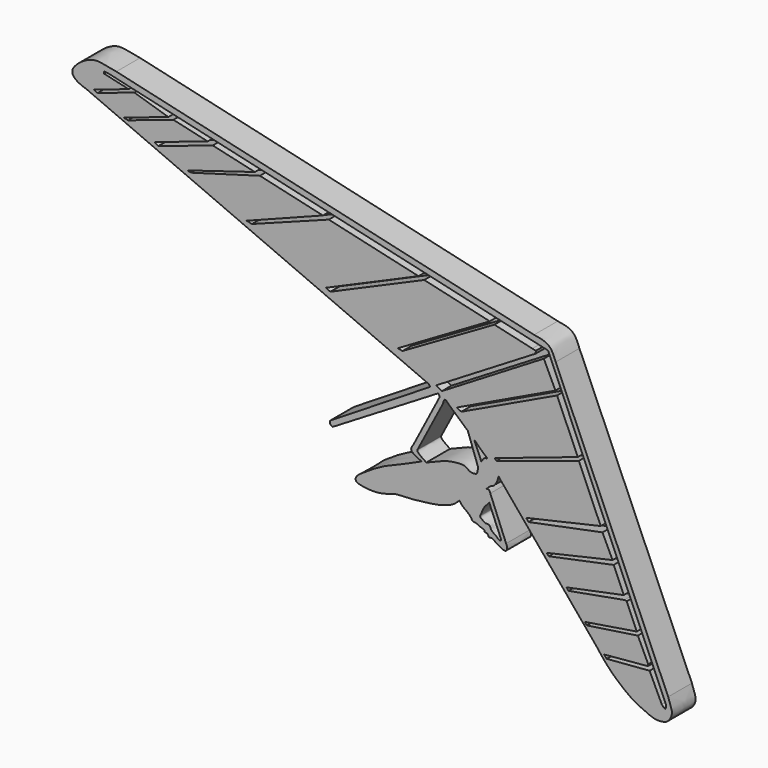
from build123d import *

# Parameters (mm, degrees)
F1_DEPTH = 3
F2_DEPTH = 5


with BuildPart() as f1:
    # F0 (on Front) → F1 (new body)
    with BuildSketch(Plane.XZ):
        with BuildLine():
            add(Edge.make_bspline(
                [(-3.958843658, -0.272790711), (-4.2719665821, 0.0142837838), (-4.643623801, 0.3451680177), (-5.0374746802, 0.6923990015)],
                knots=[0.7600893092, 0.7600893092, 0.7600893092, 0.7600893092, 0.7909645416, 0.7909645416, 0.7909645416, 0.7909645416], degree=3))
            Line((-5.0374746802, 0.6923990015), (-3.2803696069, -4.2355656273))
            add(Edge.make_bspline(
                [(-3.2803696069, -4.2355656273), (-3.1553498333, -3.8691138278), (-2.9633792204, -3.454910973), (-2.7671998453, -3.1178165413)],
                knots=[0.4986063056, 0.4986063056, 0.4986063056, 0.4986063056, 0.5447587412, 0.5447587412, 0.5447587412, 0.5447587412], degree=3))
            Line((-2.7671998453, -3.1178165413), (-3.958843658, -0.272790711))
        make_face()
    extrude(amount=F1_DEPTH)



with BuildPart() as f1b:
    # F0 (on Front) → F1, piece 2 (new body)
    with BuildSketch(Plane.XZ):
        Polygon((7.5457381318, 17.2318940768), (-65.6217709184, 34.0295992792), (-66.3976059657, 34.1109745204), (-66.3976059657, 33.7685608692), (-63.0448907614, 32.9988487065), (-62.215026468, 32.8109674156), (-68.1188135161, 30.8244369209), (-67.4496538422, 30.5345711273), (-61.2546354532, 32.6190963387), (-55.5289892554, 30.8500090748), (-63.0566432516, 28.3170731652), (-62.3126912516, 28.1462775956), (-54.6743792028, 30.7164481809), (-48.8941353204, 29.3894270209), (-57.8368790448, 26.3803359121), (-57.2307138925, 25.9741354846), (-48.0405491438, 29.066479835), (-40.9353561699, 27.43527852), (-52.3144661485, 23.9721520054), (-51.701374352, 23.8313991576), (-40.0919642747, 27.1510338508), (-29.472887516, 24.7131194919), (-42.3169331915, 19.753197379), (-41.4403453469, 19.5519514382), (-28.4778410115, 24.4221122192), (-13.3526945596, 20.9497000169), (-28.9905350655, 14.1369793564), (-28.2068449965, 13.8057659517), (-12.3952388368, 20.6941886798), (-1.3400092721, 18.1561429054), (-16.8327485305, 9.1245940536), (-16.0704851151, 8.9495945722), (-0.5562102706, 17.907858254), (5.831264226, 16.4414298492), (6.4167166129, 16.3070224226), (6.3947961883, 15.8712696639), (-10.4206494301, 5.6898728398), (-9.4167995289, 5.1668914956), (-6.9013429763, 6.6899472585), (7.7697090081, 15.5729590722), (9.7222536882, 11.4739608713), (-6.8918203924, 3.5598998321), (-6.1443895223, 3.1705065566), (10.0013106788, 10.8408021783), (13.4894661484, 2.8341303049), (-0.4957623773, -1.8716767838), (-0.2358101605, -2.1840042965), (13.6655064476, 2.3245441099), (17.3558875858, -6.1463142333), (4.8005964737, -9.0149185256), (5.2074594302, -9.5037564234), (17.6518484829, -6.989151013), (19.3531792489, -10.5476134987), (8.2439421993, -13.0858266553), (8.5738468794, -13.4822006867), (19.5388207109, -11.2054196425), (21.2328508375, -15.1317070768), (11.5879603013, -17.1178100351), (11.9304004935, -17.5292452396), (21.3820858062, -15.8089878546), (21.7298547311, -15.8888282094), (23.4441608069, -19.8238266231), (14.6837355114, -21.2355394273), (15.0275071961, -21.6485743941), (23.6202347902, -20.3643494816), (25.3650247929, -24.0533517272), (25.3243371723, -24.3517288537), (17.9191976664, -25.0162927033), (18.3667614934, -25.5181060703), (25.5955885974, -24.934917462), (27.6435296861, -29.2613615812), (28.0233658055, -29.6726883891), (28.2402802137, -29.7224873276), (28.321655455, -29.5868625463), (28.375904995, -29.1121748806), (8.4721240049, 17.0192155669), align=None)
    extrude(amount=F1_DEPTH)


with BuildPart() as f1_1:
    add(f1.part)

    add(f1b.part)  # F2 merges F1b
    # F0 (on Front) → F2 (join)
    with BuildSketch(Plane.XZ):
        with BuildLine():
            add(Edge.make_bspline(
                [(-69.2230314016, 30.4545033723), (-69.9181913826, 30.689063994), (-71.1847424521, 31.1164231839), (-72.3137756024, 32.8148190164), (-68.6665327756, 35.5511735287), (-66.3988625608, 35.128581332), (-64.9777753981, 34.86736873), (-64.2862692475, 34.7402617335)],
                knots=[0, 0, 0, 0, 0.1908374714, 0.347697523, 0.607024674, 0.8087767858, 1, 1, 1, 1], degree=3))
            Line((-69.2230314016, 30.4545033723), (-11.5922411632, 5.4900660326))
            Line((-11.5922411632, 5.4900660326), (-11.3857872784, 5.1581566222))
            Line((-11.3857872784, 5.1581566222), (-28.2431393862, -5.327432882))
            add(Edge.make_bspline(
                [(-27.8076659888, -6.1177369207), (-27.9722888528, -6.0516858021), (-28.3106523524, -5.9159252697), (-28.266044387, -5.5270896206), (-28.2431393862, -5.327432882)],
                knots=[0, 0, 0, 0, 0.4865266622, 1, 1, 1, 1], degree=3))
            Line((-27.8076659888, -6.1177369207), (-10.2219458664, 4.530044831))
            Line((-10.2219458664, 4.530044831), (-10.0369686261, 4.6426397748))
            Line((-10.0369686261, 4.6426397748), (-9.7684441134, 4.2014927603))
            Line((-9.7684441134, 4.2014927603), (-14.1773857176, -4.261362832))
            add(Edge.make_bspline(
                [(-12.7947209403, -6.3626165502), (-13.0334271505, -6.2805139246), (-13.5184917895, -6.1136767049), (-14.220189292, -5.6478018131), (-14.531709537, -5.4241327279), (-14.6556915825, -4.9871926824), (-14.3576112479, -4.5348553382), (-14.1773857176, -4.261362832)],
                knots=[0, 0, 0, 0, 0.2243166321, 0.4558241953, 0.6092440098, 0.7637408531, 1, 1, 1, 1], degree=3))
            add(Edge.make_bspline(
                [(-6.4495992847, -10.100312531), (-6.7441156637, -10.3927897932), (-7.3501218579, -10.9946002362), (-8.7041020642, -11.5541608562), (-10.0684563701, -11.9645084942), (-12.7031852773, -12.3310429211), (-15.730053764, -12.6261937319), (-17.2652343001, -12.5335072447), (-19.3279665226, -13.3871483962), (-21.2038717611, -13.4796836708), (-22.611676204, -13.359816129), (-24.0173983346, -13.0521736195), (-23.9696116255, -12.1275719541), (-22.621292381, -11.1758610844), (-21.1033539259, -10.2092903874), (-18.9497480388, -8.9271541368), (-15.0096411192, -7.423031309), (-13.4627235854, -6.6824293681), (-12.7947209403, -6.3626165502)],
                knots=[0, 0, 0, 0, 0.0512015152, 0.1053538533, 0.1595452957, 0.2346660875, 0.3143966362, 0.3709639138, 0.4378890012, 0.5004742743, 0.5561906401, 0.6069183652, 0.6431262878, 0.7002532752, 0.7618580709, 0.8346312867, 0.9285891229, 1, 1, 1, 1], degree=3))
            add(Edge.make_bspline(
                [(1.4102349523, -13.9269949868), (1.4749419549, -14.0812995688), (1.5951120677, -14.367865137), (1.6227209485, -14.8859002425), (1.1354026117, -15.1691694816), (0.4498641561, -14.7477156812), (-0.6640591092, -14.1716147874), (-0.964249599, -13.8580024095), (-1.4951999347, -14.0043591013), (-1.5685727115, -13.7207736017), (-1.8192065789, -13.3827013104), (-2.2717811663, -13.4351631175), (-2.2071364287, -13.010901004), (-2.8066379941, -13.0058014509), (-3.38081436, -12.5444686941), (-4.3147683124, -12.4988410556), (-4.4675737318, -11.9207481219), (-5.4031459263, -11.1189747582), (-5.9573777545, -10.8137728678), (-6.2798680182, -10.3410311014), (-6.4495992847, -10.100312531)],
                knots=[0, 0, 0, 0, 0.0514729921, 0.1014592787, 0.149221469, 0.2145230836, 0.2975211894, 0.3450601704, 0.3934120742, 0.4289236754, 0.47548306, 0.5189702295, 0.5567780208, 0.6075660577, 0.6723047127, 0.7388670026, 0.792399205, 0.8726835822, 0.9325882721, 1, 1, 1, 1], degree=3))
            Line((1.4102349523, -13.9269949868), (-1.2545015197, -7.343289908))
            add(Edge.make_bspline(
                [(0.4007980169, -4.7088088468), (0.310436534, -4.5520931225), (0.1140061778, -4.2114200332), (0.023724046, -5.001467346), (-0.2868815855, -5.5909447621), (-0.7107437927, -6.1131980187), (-1.2324368171, -6.2077198768), (-1.69872509, -6.6995691869), (-1.9511121659, -6.9357491466), (-1.4844889637, -6.73770814), (-1.3402720814, -7.1174467598), (-1.2545015197, -7.343289908)],
                knots=[0, 0, 0, 0, 0.0984772063, 0.2140725462, 0.3524954365, 0.4780678856, 0.5924230264, 0.7267704517, 0.7940044635, 0.8774876243, 1, 1, 1, 1], degree=3))
            Line((0.4007980169, -4.7088088468), (16.64548181, -24.2264792323))
            add(Edge.make_bspline(
                [(28.7290737033, -27.7940165251), (28.9117644633, -28.3099578967), (29.2391090465, -29.2344196111), (29.4945885215, -30.1956884574), (28.7931095169, -31.4654049104), (28.0013465038, -31.7902524263), (26.5785107763, -31.9730053275), (24.6056557437, -31.0893777432), (22.4111262769, -30.1005694812), (18.7903829231, -27.053984243), (17.329002501, -25.1275269155), (16.64548181, -24.2264792323)],
                knots=[0, 0, 0, 0, 0.0993022054, 0.1779293, 0.2692963707, 0.341902863, 0.4346793497, 0.5499136078, 0.6756716751, 0.8483043037, 1, 1, 1, 1], degree=3))
            Line((28.7290737033, -27.7940165251), (9.7696268931, 15.7252792269))
            add(Edge.make_bspline(
                [(6.1201294884, 18.5764487833), (6.794057073, 18.470796703), (8.0256136154, 18.2777247564), (9.1324021938, 17.3905574188), (9.5470495227, 16.3069472653), (9.7696268931, 15.7252792269)],
                knots=[0, 0, 0, 0, 0.3589004256, 0.6558659674, 1, 1, 1, 1], degree=3))
            Line((6.1201294884, 18.5764487833), (-64.2862692475, 34.7402617335))
        make_face()
        with BuildLine():
            add(Edge.make_bspline(
                [(0.4983769031, -13.4383020923), (0.5218137706, -13.5645244168), (0.5644444565, -13.7941175684), (0.2328431432, -13.8910706937), (-0.1654042371, -13.3790911879), (-0.7574425902, -13.0664055933), (-1.2446881019, -12.6109943897), (-1.3271120749, -11.9540819736), (-2.10476145, -12.1123359576), (-2.3607071265, -11.8356934552), (-3.1441042369, -11.4224284839), (-2.6973194121, -10.7189183877), (-2.3203517948, -9.7046953475), (-1.857624161, -9.2747417349), (-1.5794103674, -8.9316595418), (-1.4388341224, -8.7583065033)],
                knots=[0, 0, 0, 0, 0.0576076042, 0.1047858328, 0.1828799237, 0.2674298299, 0.3488641516, 0.4218594737, 0.5010696502, 0.5644708288, 0.6493186164, 0.7324956406, 0.8386246949, 0.9184600658, 1, 1, 1, 1], degree=3))
            Line((-1.4388341224, -8.7583065033), (0.4983769031, -13.4383020923))
        make_face(mode=Mode.SUBTRACT)
        with BuildLine():
            Line((-13.5296313092, -4.8642060719), (-9.2414719984, 3.3471633215))
            add(Edge.make_bspline(
                [(-5.0374746802, 0.6923990015), (-6.2098649377, 1.7260141184), (-8.2743854108, 3.5031337653), (-8.6626945193, 4.0403415153), (-9.0047233819, 4.1212678088), (-9.1342331249, 3.692152472), (-9.2414719984, 3.3471633215)],
                knots=[0.7909645416, 0.7909645416, 0.7909645416, 0.7909645416, 0.8828719703, 0.9295607436, 0.9530977505, 1, 1, 1, 1], degree=3))
            add(Edge.make_bspline(
                [(-3.958843658, -0.272790711), (-4.2719665821, 0.0142837838), (-4.643623801, 0.3451680177), (-5.0374746802, 0.6923990015)],
                knots=[0.7600893092, 0.7600893092, 0.7600893092, 0.7600893092, 0.7909645416, 0.7909645416, 0.7909645416, 0.7909645416], degree=3))
            add(Edge.make_bspline(
                [(-2.7671998453, -3.1178165413), (-2.7186353622, -3.0343683356), (-2.4670899427, -2.6287681187), (-2.1264112601, -2.2928308378), (-1.557684599, -2.4383425244), (-2.5904654003, -1.6700994255), (-3.0885284809, -1.077271621), (-3.8801984268, -0.3448935124), (-3.958843658, -0.272790711)],
                knots=[0.5447587412, 0.5447587412, 0.5447587412, 0.5447587412, 0.5561838422, 0.603623763, 0.6307813896, 0.6781816144, 0.7523345599, 0.7600893092, 0.7600893092, 0.7600893092, 0.7600893092], degree=3))
            add(Edge.make_bspline(
                [(-3.2803696069, -4.2355656273), (-3.1553498333, -3.8691138278), (-2.9633792204, -3.454910973), (-2.7671998453, -3.1178165413)],
                knots=[0.4986063056, 0.4986063056, 0.4986063056, 0.4986063056, 0.5447587412, 0.5447587412, 0.5447587412, 0.5447587412], degree=3))
            add(Edge.make_bspline(
                [(-12.0408171788, -6.2805139246), (-11.5311187477, -6.0578584946), (-10.7086710037, -5.6985898211), (-9.4370105372, -5.1885311265), (-8.3247583539, -4.8296994289), (-6.7493021945, -4.5824676231), (-5.4959904023, -4.609683443), (-4.9454383959, -5.0427472099), (-4.7396669328, -5.2771718305), (-3.4292763562, -5.3943179608), (-3.454698522, -4.8096858391), (-3.3214686036, -4.3560329811), (-3.2803696069, -4.2355656273)],
                knots=[0, 0, 0, 0, 0.0652530186, 0.1265638703, 0.1845710832, 0.2524331328, 0.3120420087, 0.3537084073, 0.3842297899, 0.4389143927, 0.4834341552, 0.4986063056, 0.4986063056, 0.4986063056, 0.4986063056], degree=3))
            add(Edge.make_bspline(
                [(-13.5296313092, -4.8642060719), (-13.5517841798, -4.9326845236), (-13.6378246412, -5.1986508486), (-12.7213366532, -5.8195086324), (-12.0408171788, -6.2805139246)],
                knots=[0, 0, 0, 0, 0.2574703833, 1, 1, 1, 1], degree=3))
        make_face(mode=Mode.SUBTRACT)
        Polygon((-66.3976059657, 34.1109745204), (-65.6217709184, 34.0295992792), (7.5457381318, 17.2318940768), (8.4721240049, 17.0192155669), (28.375904995, -29.1121748806), (28.321655455, -29.5868625463), (28.2402802137, -29.7224873276), (28.0233658055, -29.6726883891), (27.6435296861, -29.2613615812), (25.5955885974, -24.934917462), (18.3667614934, -25.5181060703), (17.9191976664, -25.0162927033), (25.3243371723, -24.3517288537), (25.3650247929, -24.0533517272), (23.6202347902, -20.3643494816), (15.0275071961, -21.6485743941), (14.6837355114, -21.2355394273), (23.4441608069, -19.8238266231), (21.7298547311, -15.8888282094), (21.3820858062, -15.8089878546), (11.9304004935, -17.5292452396), (11.5879603013, -17.1178100351), (21.2328508375, -15.1317070768), (19.5388207109, -11.2054196425), (8.5738468794, -13.4822006867), (8.2439421993, -13.0858266553), (19.3531792489, -10.5476134987), (17.6518484829, -6.989151013), (5.2074594302, -9.5037564234), (4.8005964737, -9.0149185256), (17.3558875858, -6.1463142333), (13.6655064476, 2.3245441099), (-0.2358101605, -2.1840042965), (-0.4957623773, -1.8716767838), (13.4894661484, 2.8341303049), (10.0013106788, 10.8408021783), (-6.1443895223, 3.1705065566), (-6.8918203924, 3.5598998321), (9.7222536882, 11.4739608713), (7.7697090081, 15.5729590722), (-6.9013429763, 6.6899472585), (-9.4167995289, 5.1668914956), (-10.4206494301, 5.6898728398), (6.3947961883, 15.8712696639), (6.4167166129, 16.3070224226), (5.831264226, 16.4414298492), (-0.5562102706, 17.907858254), (-16.0704851151, 8.9495945722), (-16.8327485305, 9.1245940536), (-1.3400092721, 18.1561429054), (-12.3952388368, 20.6941886798), (-28.2068449965, 13.8057659517), (-28.9905350655, 14.1369793564), (-13.3526945596, 20.9497000169), (-28.4778410115, 24.4221122192), (-41.4403453469, 19.5519514382), (-42.3169331915, 19.753197379), (-29.472887516, 24.7131194919), (-40.0919642747, 27.1510338508), (-51.701374352, 23.8313991576), (-52.3144661485, 23.9721520054), (-40.9353561699, 27.43527852), (-48.0405491438, 29.066479835), (-57.2307138925, 25.9741354846), (-57.8368790448, 26.3803359121), (-48.8941353204, 29.3894270209), (-54.6743792028, 30.7164481809), (-62.3126912516, 28.1462775956), (-63.0566432516, 28.3170731652), (-55.5289892554, 30.8500090748), (-61.2546354532, 32.6190963387), (-67.4496538422, 30.5345711273), (-68.1188135161, 30.8244369209), (-62.215026468, 32.8109674156), (-63.0448907614, 32.9988487065), (-66.3976059657, 33.7685608692), align=None, mode=Mode.SUBTRACT)
        with BuildLine():
            add(Edge.make_bspline(
                [(-3.958843658, -0.272790711), (-4.2719665821, 0.0142837838), (-4.643623801, 0.3451680177), (-5.0374746802, 0.6923990015)],
                knots=[0.7600893092, 0.7600893092, 0.7600893092, 0.7600893092, 0.7909645416, 0.7909645416, 0.7909645416, 0.7909645416], degree=3))
            Line((-5.0374746802, 0.6923990015), (-3.2803696069, -4.2355656273))
            add(Edge.make_bspline(
                [(-3.2803696069, -4.2355656273), (-3.1553498333, -3.8691138278), (-2.9633792204, -3.454910973), (-2.7671998453, -3.1178165413)],
                knots=[0.4986063056, 0.4986063056, 0.4986063056, 0.4986063056, 0.5447587412, 0.5447587412, 0.5447587412, 0.5447587412], degree=3))
            Line((-2.7671998453, -3.1178165413), (-3.958843658, -0.272790711))
        make_face()
    extrude(amount=F2_DEPTH)


solid = f1_1.part
